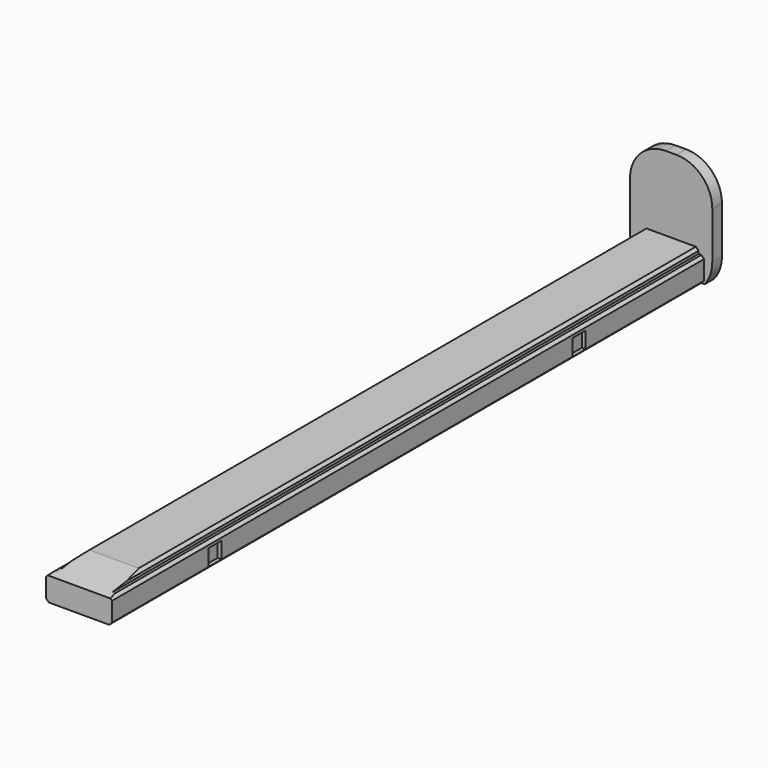
from build123d import *

# Parameters (mm, degrees)
F1_DEPTH = 135
F2_SIZE2 = 8
F2_SIZE  = 1.2
F4_DEPTH = 2.2
F5_W     = 3
F5_H     = 3
F6_DEPTH = 0.7
F7_SIZE  = 0.49999
F8_W     = 4.2
F8_H     = 130.6
F9_DEPTH = 4
F10_SIZE = 1


# Not quite as in the source:
# - a fillet or chamfer is up to 0.001 mm smaller than in the source, because OpenCascade refuses the exact size
# - a pattern or mirror of a feature is missing from the dataset's text; its kind, count and spacing are read off the source's solid


with BuildPart() as f1:
    # F0 (on Front) → F1 (new body)
    with BuildSketch(Plane.XZ):
        Polygon((-6, -2.75), (6, -2.75), (6, 1.75), (5, 1.75), (5, 2.75), (-5, 2.75), (-5, 1.75), (-6, 1.75), align=None)
    extrude(amount=F1_DEPTH)

    # F2
    f2_edges = [f1.edges().sort_by_distance(p)[0] for p in [
        (0, -135, 2.75),
    ]]
    f2_side = f1.faces().sort_by_distance((0, -135, -0.070312))[0]
    chamfer(f2_edges, length=F2_SIZE, length2=F2_SIZE2, reference=f2_side)

    # F3 (on Front) → F4 (join)
    with BuildSketch(Plane.XZ):
        with BuildLine():
            ThreePointArc((7.5, 9.85), (5.5961940777, 14.4461940777), (1, 16.35))
            Line((1, 16.35), (-1, 16.35))
            ThreePointArc((-1, 16.35), (-5.5961940777, 14.4461940777), (-7.5, 9.85))
            Line((-7.5, 9.85), (-7.5, 1.25))
            ThreePointArc((-7.5, 1.25), (-7.1462423475, -0.8651134734), (-6.123475383, -2.75))
            Line((-6.123475383, -2.75), (6.123475383, -2.75))
            ThreePointArc((6.123475383, -2.75), (7.1462423475, -0.8651134734), (7.5, 1.25))
            Line((7.5, 1.25), (7.5, 9.85))
        make_face()
    extrude(amount=-F4_DEPTH)

    # F5 (on face) → F6 (cut)
    with BuildSketch(Plane(origin=(-6, 0, 0), x_dir=(0, -1, 0), z_dir=(-1, 0, 0))):
        with Locations((28.5, -0.75)):
            Rectangle(F5_W, F5_H)
        with Locations((111.5, -0.75)):
            Rectangle(F5_W, F5_H)
    f6 = extrude(amount=-F6_DEPTH, mode=Mode.SUBTRACT)

    # F6_copies: F6 across plane
    add(f6.mirror(Plane(origin=(0, 0, 0), x_dir=(0, 0, 1), z_dir=(1, 0, 0))), mode=Mode.SUBTRACT)

    # F7 (size 0.5 in the source; OpenCascade refuses exactly that, so slightly less here)
    f7_edges = [f1.edges().sort_by_distance(p)[0] for p in [
        (6, -67.5, -2.75),
        (-6, -67.5, -2.75),
        (6, -66.833333, 1.75),
        (5, -63.5, 2.75),
        (-5, -63.5, 2.75),
        (-6, -66.833333, 1.75),
    ]]
    chamfer(f7_edges, length=F7_SIZE)

    # F8 (on face) → F9 (cut)
    with BuildSketch(Plane(origin=(0, 0, -2.75), x_dir=(1, 0, 0), z_dir=(0, 0, -1))):
        with Locations((0, 67.5)):
            Rectangle(F8_W, F8_H)
    extrude(amount=-F9_DEPTH, mode=Mode.SUBTRACT)

    # F10
    f10_edges = [f1.edges().sort_by_distance(p)[0] for p in [
        (0, -132.8, 1.25),
        (-2.1, -67.5, 1.25),
        (2.1, -67.5, 1.25),
        (0, -2.2, 1.25),
        (2.1, -67.5, -2.75),
        (-2.1, -67.5, -2.75),
    ]]
    chamfer(f10_edges, length=F10_SIZE)


solid = f1.part
